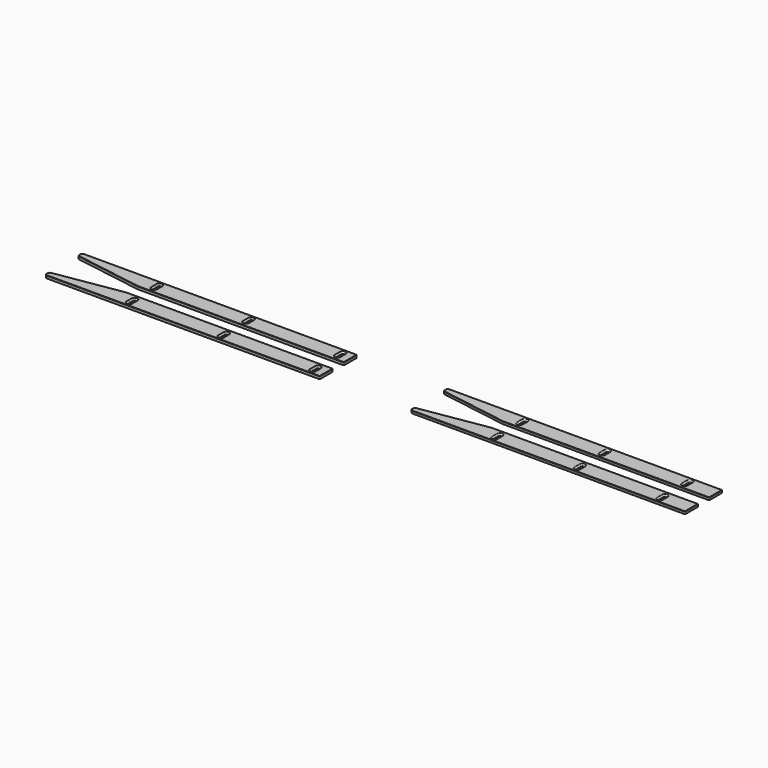
from build123d import *

# Parameters (mm, degrees)
F1_DEPTH      = 3
F4_R          = 3
F4_2_R        = 3
F6_R          = 1
F6_2_R        = 1
F7_SIZE       = 0.3
F7_2_SIZE     = 0.3
F8_SIZE2      = 1.7
F8_SIZE       = 1.7
F8_2_SIZE2    = 1.7
F8_2_SIZE     = 1.7
F10_DEPTH     = 2.7
F11_R         = 3
F12_SIZE2     = 1.7
F12_SIZE      = 1.7
F13_R         = 1
F14_T1_DEPTH  = 296
F14_T3_DEPTH  = 16
F14_T5_DEPTH  = 0.2959256647
F14_T7_DEPTH  = 226.2787712738
F14_T9_DEPTH  = 75.7744230165
F14_T11_DEPTH = 7
F14_T14_ANGLE = 90
F14_T16_ANGLE = 90
F14_T18_ANGLE = 90
F14_T20_ANGLE = 80.8017433596
F14_T22_ANGLE = 180
F14_T24_ANGLE = 180
F14_T26_ANGLE = 180
F14_T28_ANGLE = 180
F14_T30_ANGLE = 180
F14_T32_ANGLE = 180


# Not quite as in the source:
# - a fillet or chamfer that OpenCascade refuses, or shapes differently, is made with other operations: its cross-section is extruded or revolved along the edge and cut away or added
# - two fillets or chamfers of one size are made in one step
# - a feature names something its author has since deleted; it is built from what else it names


with BuildPart() as f1:
    # F0 (on Top) → F1 (new body)
    with BuildSketch(Plane.XY):
        Polygon((0, 5.8492044918), (0, 0), (300, 0), (300, 18), (75.0357434154, 18), align=None)
        with BuildLine():
            Line((89.974817574, 12), (89.974817574, 5))
            ThreePointArc((89.974817574, 5), (88.474817574, 3.5), (86.974817574, 5))
            Line((86.974817574, 5), (86.974817574, 12))
            ThreePointArc((86.974817574, 12), (88.474817574, 13.5), (89.974817574, 12))
        make_face(mode=Mode.SUBTRACT)
        with BuildLine():
            Line((189.974817574, 12), (189.974817574, 5))
            ThreePointArc((189.974817574, 5), (188.474817574, 3.5), (186.974817574, 5))
            Line((186.974817574, 5), (186.974817574, 12))
            ThreePointArc((186.974817574, 12), (188.474817574, 13.5), (189.974817574, 12))
        make_face(mode=Mode.SUBTRACT)
        with BuildLine():
            Line((289.974817574, 12), (289.974817574, 5))
            ThreePointArc((289.974817574, 5), (288.474817574, 3.5), (286.974817574, 5))
            Line((286.974817574, 5), (286.974817574, 12))
            ThreePointArc((286.974817574, 12), (288.474817574, 13.5), (289.974817574, 12))
        make_face(mode=Mode.SUBTRACT)
    extrude(amount=F1_DEPTH)


with BuildPart() as f3_1:
    # F3: instance of F1
    add(f1.part.mirror(Plane(origin=(150, 25.4, 1.5), x_dir=(1, 0, 0), z_dir=(0, -1, 0))))

    # F4#2
    f4_2_edges = [f3_1.edges().sort_by_distance(p)[0] for p in [
        (0, 44.950796, 1.5),
        (0, 50.8, 1.5),
    ]]
    fillet(f4_2_edges, radius=F4_2_R)

    # F6#2
    f6_2_edges = [f3_1.edges().sort_by_distance(p)[0] for p in [
        (300, 50.8, 1.5),
        (300, 32.8, 1.5),
    ]]
    fillet(f6_2_edges, radius=F6_2_R)

    # F7#2
    f7_2_edges = [f3_1.edges().sort_by_distance(p)[0] for p in [
        (187.017872, 32.8, 3),
    ]]
    chamfer(f7_2_edges, length=F7_2_SIZE)

    # F8#2
    f8_2_edges = [f3_1.edges().sort_by_distance(p)[0] for p in [
        (189.974818, 42.3, 3),
        (188.474818, 37.3, 3),
        (186.974818, 42.3, 3),
        (188.474818, 47.3, 3),
        (88.474818, 47.3, 3),
        (89.974818, 42.3, 3),
        (88.474818, 37.3, 3),
        (86.974818, 42.3, 3),
        (289.974818, 42.3, 3),
        (286.974818, 42.3, 3),
        (288.474818, 47.3, 3),
        (288.474818, 37.3, 3),
    ]]
    chamfer(f8_2_edges, length=F8_2_SIZE, length2=F8_2_SIZE2)


with BuildPart() as f1_1:
    add(f1.part)

    # F4
    f4_edges = [f1_1.edges().sort_by_distance(p)[0] for p in [
        (0, 5.849204, 1.5),
        (0, 0, 1.5),
    ]]
    fillet(f4_edges, radius=F4_R)

    # F6
    f6_edges = [f1_1.edges().sort_by_distance(p)[0] for p in [
        (300, 0, 1.5),
        (300, 18, 1.5),
    ]]
    fillet(f6_edges, radius=F6_R)

    # F7
    f7_edges = [f1_1.edges().sort_by_distance(p)[0] for p in [
        (187.017872, 18, 3),
    ]]
    chamfer(f7_edges, length=F7_SIZE)

    # F8
    f8_edges = [f1_1.edges().sort_by_distance(p)[0] for p in [
        (89.974818, 8.5, 3),
        (88.474818, 13.5, 3),
        (86.974818, 8.5, 3),
        (88.474818, 3.5, 3),
        (188.474818, 13.5, 3),
        (189.974818, 8.5, 3),
        (188.474818, 3.5, 3),
        (186.974818, 8.5, 3),
        (289.974818, 8.5, 3),
        (288.474818, 13.5, 3),
        (288.474818, 3.5, 3),
        (286.974818, 8.5, 3),
    ]]
    chamfer(f8_edges, length=F8_SIZE, length2=F8_SIZE2)


with BuildPart() as f10:
    # F9 (on face) → F10 (new body)
    with BuildSketch(Plane(origin=(0, 0, 0), x_dir=(1, 0, 0), z_dir=(0, 0, -1))):
        Polygon((398.4068919917, -45.0014215894), (398.4068919917, -50.8506260812), (698.4068919917, -50.8506260812), (698.4068919917, -32.8506260812), (473.4426354071, -32.8506260812), align=None)
        with BuildLine():
            Line((488.3817095657, -38.8506260812), (488.3817095657, -45.8506260812))
            ThreePointArc((488.3817095657, -45.8506260812), (486.8817095657, -47.3506260812), (485.3817095657, -45.8506260812))
            Line((485.3817095657, -45.8506260812), (485.3817095657, -38.8506260812))
            ThreePointArc((485.3817095657, -38.8506260812), (486.8817095657, -37.3506260812), (488.3817095657, -38.8506260812))
        make_face(mode=Mode.SUBTRACT)
        with BuildLine():
            Line((578.3817095657, -38.8506260812), (578.3817095657, -45.8506260812))
            ThreePointArc((578.3817095657, -45.8506260812), (576.8817095657, -47.3506260812), (575.3817095657, -45.8506260812))
            Line((575.3817095657, -45.8506260812), (575.3817095657, -38.8506260812))
            ThreePointArc((575.3817095657, -38.8506260812), (576.8817095657, -37.3506260812), (578.3817095657, -38.8506260812))
        make_face(mode=Mode.SUBTRACT)
        with BuildLine():
            Line((668.3817095657, -38.8506260812), (668.3817095657, -45.8506260812))
            ThreePointArc((668.3817095657, -45.8506260812), (666.8817095657, -47.3506260812), (665.3817095657, -45.8506260812))
            Line((665.3817095657, -45.8506260812), (665.3817095657, -38.8506260812))
            ThreePointArc((665.3817095657, -38.8506260812), (666.8817095657, -37.3506260812), (668.3817095657, -38.8506260812))
        make_face(mode=Mode.SUBTRACT)
    extrude(amount=-F10_DEPTH)

    # F11
    f11_edges = [f10.edges().sort_by_distance(p)[0] for p in [
        (398.406892, 45.001422, 1.35),
        (398.406892, 50.850626, 1.35),
    ]]
    fillet(f11_edges, radius=F11_R)

    # F12
    f12_edges = [f10.edges().sort_by_distance(p)[0] for p in [
        (486.88171, 47.350626, 2.7),
        (485.38171, 42.350626, 2.7),
        (488.38171, 42.350626, 2.7),
        (486.88171, 37.350626, 2.7),
        (575.38171, 42.350626, 2.7),
        (576.88171, 47.350626, 2.7),
        (578.38171, 42.350626, 2.7),
        (576.88171, 37.350626, 2.7),
        (665.38171, 42.350626, 2.7),
        (668.38171, 42.350626, 2.7),
        (666.88171, 47.350626, 2.7),
        (666.88171, 37.350626, 2.7),
    ]]
    chamfer(f12_edges, length=F12_SIZE, length2=F12_SIZE2)

    # F13
    f13_edges = [f10.edges().sort_by_distance(p)[0] for p in [
        (698.406892, 32.850626, 1.35),
        (698.406892, 50.850626, 1.35),
    ]]
    fillet(f13_edges, radius=F13_R)

    # F14: chamfer of 0.3 on 21 edges, made by hand

    # F14_s2 → F14_t1 (cut)
    with BuildSketch(Plane.YZ.offset(401.4068919917)):
        Polygon((50.5506260812, 2.7), (50.8506260812, 2.4), (50.8506260812, 2.7), align=None)
    extrude(amount=F14_T1_DEPTH, mode=Mode.SUBTRACT)

    # F14_s4 → F14_t3 (cut)
    with BuildSketch(Plane.XZ.offset(-49.8506260812)):
        Polygon((698.1068919917, 2.7), (698.4068919917, 2.4), (698.4068919917, 2.7), align=None)
    extrude(amount=F14_T3_DEPTH, mode=Mode.SUBTRACT)

    # F14_s6 → F14_t5 (cut)
    with BuildSketch(Plane.XZ.offset(-47.8506260812)):
        Polygon((398.7068919917, 2.7), (398.4068919917, 2.4), (398.4068919917, 2.7), align=None)
    extrude(amount=F14_T5_DEPTH, mode=Mode.SUBTRACT)

    # F14_s8 → F14_t7 (cut)
    with BuildSketch(Plane.YZ.offset(471.1281207179)):
        Polygon((33.1506260812, 2.7), (32.8506260812, 2.4), (32.8506260812, 2.7), align=None)
    extrude(amount=F14_T7_DEPTH, mode=Mode.SUBTRACT)

    # F14_s10 → F14_t9 (cut)
    with BuildSketch(Plane(origin=(458.4461110865, -74.2377524868, 0), x_dir=(0, 0, 1), z_dir=(-0.9871411294, 0.1598511517, 0))):
        Polygon((2.7, 108.4085546466), (2.4, 108.1085546466), (2.7, 108.1085546466), align=None)
    extrude(amount=F14_T9_DEPTH, mode=Mode.SUBTRACT)

    # F14_s12 → F14_t11 (cut)
    with BuildSketch(Plane.XZ.offset(-45.8506260812)):
        Polygon((490.2059736344, 2.7), (489.9938416001, 2.6121320344), (490.0817095657, 2.7), align=None)
        Polygon((483.557445497, 2.7), (483.7695775314, 2.6121320344), (483.6817095657, 2.7), align=None)
        Polygon((573.557445497, 2.7), (573.7695775314, 2.6121320344), (573.6817095657, 2.7), align=None)
        Polygon((580.2059736344, 2.7), (579.9938416001, 2.6121320344), (580.0817095657, 2.7), align=None)
        Polygon((663.557445497, 2.7), (663.7695775314, 2.6121320344), (663.6817095657, 2.7), align=None)
        Polygon((670.2059736344, 2.7), (669.9938416001, 2.6121320344), (670.0817095657, 2.7), align=None)
    extrude(amount=F14_T11_DEPTH, mode=Mode.SUBTRACT)

    # F14_s13 → F14_t14 (revolve, cut)
    with BuildSketch(Plane.YZ.offset(697.4068919917)):
        Polygon((50.5506260812, 2.7), (50.8506260812, 2.4), (50.8506260812, 2.7), align=None)
    revolve(axis=Axis((697.4068919917, 49.8506260812, 2.7), (0, 0, -1)), revolution_arc=F14_T14_ANGLE, mode=Mode.SUBTRACT)

    # F14_s15 → F14_t16 (revolve, cut)
    with BuildSketch(Plane.XZ.offset(-47.8506260812)):
        Polygon((398.7068919917, 2.7), (398.4068919917, 2.4), (398.4068919917, 2.7), align=None)
    revolve(axis=Axis((401.4068919917, 47.8506260812, 2.7), (0, 0, -1)), revolution_arc=F14_T16_ANGLE, mode=Mode.SUBTRACT)

    # F14_s17 → F14_t18 (revolve, cut)
    with BuildSketch(Plane.YZ.offset(697.4068919917)):
        Polygon((33.1506260812, 2.7), (32.8506260812, 2.4), (32.8506260812, 2.7), align=None)
    revolve(axis=Axis((697.4068919917, 33.8506260812, 2.7), (0, 0, 1)), revolution_arc=F14_T18_ANGLE, mode=Mode.SUBTRACT)

    # F14_s19 → F14_t20 (revolve, cut)
    with BuildSketch(Plane.XZ.offset(-47.5547004165)):
        Polygon((398.7068919917, 2.7), (398.4068919917, 2.4), (398.4068919917, 2.7), align=None)
    revolve(axis=Axis((401.4068919917, 47.5547004165, 2.7), (0, 0, 1)), revolution_arc=F14_T20_ANGLE, mode=Mode.SUBTRACT)

    # F14_s21 → F14_t22 (revolve, cut)
    with BuildSketch(Plane.XZ.offset(-45.8506260812)):
        Polygon((490.2059736344, 2.7), (489.9938416001, 2.6121320344), (490.0817095657, 2.7), align=None)
    revolve(axis=Axis((486.8817095657, 45.8506260812, 2.7), (0, 0, 1)), revolution_arc=F14_T22_ANGLE, mode=Mode.SUBTRACT)

    # F14_s23 → F14_t24 (revolve, cut)
    with BuildSketch(Plane.XZ.offset(-38.8506260812)):
        Polygon((483.557445497, 2.7), (483.7695775314, 2.6121320344), (483.6817095657, 2.7), align=None)
    revolve(axis=Axis((486.8817095657, 38.8506260812, 2.7), (0, 0, 1)), revolution_arc=F14_T24_ANGLE, mode=Mode.SUBTRACT)

    # F14_s25 → F14_t26 (revolve, cut)
    with BuildSketch(Plane.XZ.offset(-45.8506260812)):
        Polygon((580.2059736344, 2.7), (579.9938416001, 2.6121320344), (580.0817095657, 2.7), align=None)
    revolve(axis=Axis((576.8817095657, 45.8506260812, 2.7), (0, 0, 1)), revolution_arc=F14_T26_ANGLE, mode=Mode.SUBTRACT)

    # F14_s27 → F14_t28 (revolve, cut)
    with BuildSketch(Plane.XZ.offset(-38.8506260812)):
        Polygon((573.557445497, 2.7), (573.7695775314, 2.6121320344), (573.6817095657, 2.7), align=None)
    revolve(axis=Axis((576.8817095657, 38.8506260812, 2.7), (0, 0, 1)), revolution_arc=F14_T28_ANGLE, mode=Mode.SUBTRACT)

    # F14_s29 → F14_t30 (revolve, cut)
    with BuildSketch(Plane.XZ.offset(-45.8506260812)):
        Polygon((670.2059736344, 2.7), (669.9938416001, 2.6121320344), (670.0817095657, 2.7), align=None)
    revolve(axis=Axis((666.8817095657, 45.8506260812, 2.7), (0, 0, 1)), revolution_arc=F14_T30_ANGLE, mode=Mode.SUBTRACT)

    # F14_s31 → F14_t32 (revolve, cut)
    with BuildSketch(Plane.XZ.offset(-38.8506260812)):
        Polygon((663.557445497, 2.7), (663.7695775314, 2.6121320344), (663.6817095657, 2.7), align=None)
    revolve(axis=Axis((666.8817095657, 38.8506260812, 2.7), (0, 0, 1)), revolution_arc=F14_T32_ANGLE, mode=Mode.SUBTRACT)


with BuildPart() as f15_1:
    # F15: instance of F10
    add(f10.part.mirror(Plane(origin=(150, 25.4, 1.5), x_dir=(1, 0, 0), z_dir=(0, -1, 0))))


solid = Compound([f3_1.part, f1_1.part, f10.part, f15_1.part])
